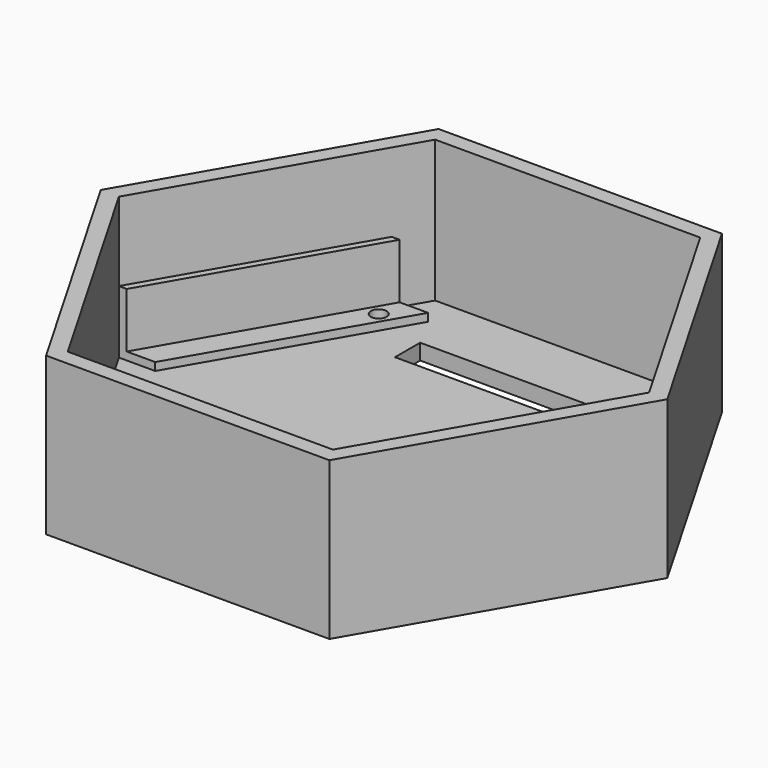
from build123d import *

# Parameters (mm, degrees)
F1_DEPTH = 3.175
F2_W     = 39.2063558102
F2_H     = 6.35
F3_DEPTH = 25.4
F4_DEPTH = 31.75
F6_DEPTH = 12.7
F7_DEPTH = 1.5875
F8_R     = 1.5875
F9_DEPTH = 25.4


# Not quite as in the source:
# - a pattern or mirror of a feature is missing from the dataset's text; its kind, count and spacing are read off the source's solid


with BuildPart() as f1:
    # F0 (on Top) → F1 (new body)
    with BuildSketch(Plane.XY):
        Polygon((-26.7419128953, 46.3183518263), (-53.4838257906, 0), (-26.7419128953, -46.3183518263), (26.7419128953, -46.3183518263), (53.4838257906, 0), (26.7419128953, 46.3183518263), align=None)
    extrude(amount=F1_DEPTH)

    # F2 (on face) → F3 (cut)
    with BuildSketch(Plane.XY.offset(3.175)):
        with Locations((0, -30.4433518263)):
            Rectangle(F2_W, F2_H)
    f3 = extrude(amount=-F3_DEPTH, mode=Mode.SUBTRACT)

    # F3_copies: F3 across plane
    add(f3.mirror(Plane.ZX), mode=Mode.SUBTRACT)


with BuildPart() as f4:
    # F0 (on Top) → F4 (new body)
    with BuildSketch(Plane.XY):
        Polygon((28.575, 49.4933518263), (-28.575, 49.4933518263), (-57.15, 0), (-28.575, -49.4933518263), (28.575, -49.4933518263), (57.15, 0), align=None)
        Polygon((-26.7419128953, -46.3183518263), (-53.4838257906, 0), (-26.7419128953, 46.3183518263), (26.7419128953, 46.3183518263), (53.4838257906, 0), (26.7419128953, -46.3183518263), align=None, mode=Mode.SUBTRACT)
    extrude(amount=F4_DEPTH)


with BuildPart() as f6:
    # F5 (on face) → F6 (new body)
    with BuildSketch(Plane.XY.offset(3.175)):
        Polygon((-51.8963257906, 0), (-28.8205871047, 39.9683518263), (-30.4080871047, 39.9683518263), (-53.4838257906, 0), align=None)
    extrude(amount=F6_DEPTH)

    # F5 (on face) → F7 (join)
    with BuildSketch(Plane.XY.offset(3.175)):
        Polygon((-46.1514773719, 0), (-23.075738686, 39.9683518263), (-28.8205871047, 39.9683518263), (-51.8963257906, 0), align=None)
    extrude(amount=F7_DEPTH)


with BuildPart() as f9_tool:
    # F8 (on face) → F9 (new body)
    with BuildSketch(Plane.XY.offset(4.7625)):
        with Locations((-28.9196960247, 34.8182901413)):
            Circle(F8_R)
    extrude(amount=-F9_DEPTH)


with BuildPart() as f1_1:
    add(f1.part)

    # F9: cut by f9_tool
    add(f9_tool.part, mode=Mode.SUBTRACT)


with BuildPart() as f6_1:
    add(f6.part)

    # F9: cut by f9_tool
    add(f9_tool.part, mode=Mode.SUBTRACT)


solid = Compound([f4.part, f1_1.part, f6_1.part])
